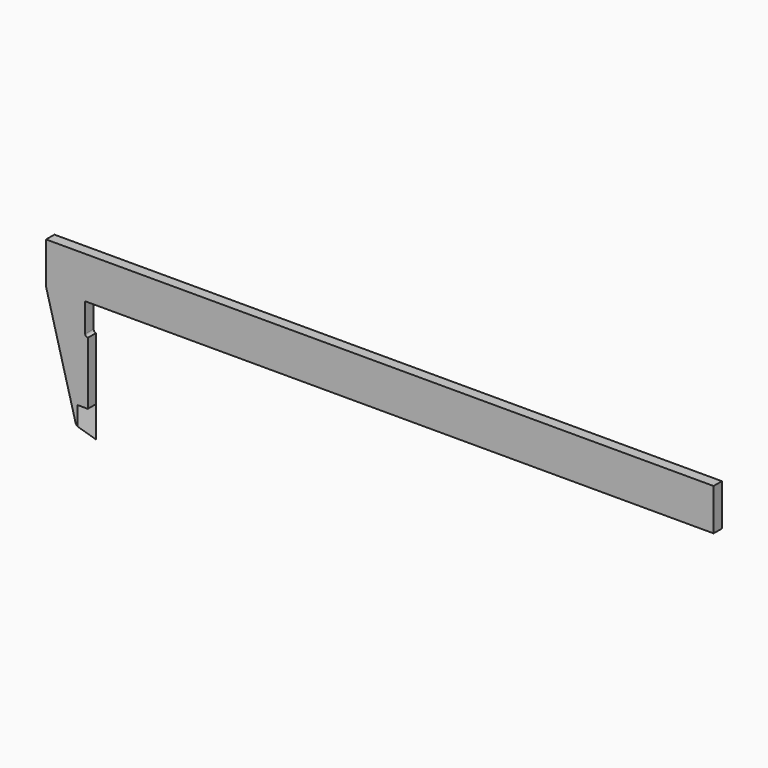
from build123d import *

# Parameters (mm, degrees)
F1_DEPTH = 3.175
F3_DEPTH = 9.525
F5_DEPTH = 3.176


# Not quite as in the source:
# - a feature names something its author has since deleted; it is built from what else it names


with BuildPart() as f1:
    # F0 (on Front) → F1 (new body)
    with BuildSketch(Plane.XZ):
        with BuildLine():
            Line((101.6, 6.35), (-101.6, 6.35))
            Line((-101.6, 6.35), (-101.6, -6.35))
            Line((-101.6, -6.35), (-92.5598257878, -40.0883894691))
            Line((-92.5598257878, -40.0883894691), (-92.075, -40.6661823435))
            Line((-92.075, -40.6661823435), (-92.075, -34.925))
            Line((-92.075, -34.925), (-88.9, -34.925))
            Line((-88.9, -34.925), (-88.9, -15.875))
            ThreePointArc((-88.9, -15.875), (-89.4567758795, -15.6443758795), (-89.6874, -15.0876))
            Line((-89.6874, -15.0876), (-89.6874, -6.35))
            Line((-89.6874, -6.35), (101.6, -6.35))
            Line((101.6, -6.35), (101.6, 6.35))
        make_face()
    extrude(amount=F1_DEPTH)

    # F2 (on face) → F3 (join)
    with BuildSketch(Plane(origin=(0, 0, -34.925), x_dir=(1, 0, 0), z_dir=(0, 0, -1))):
        Polygon((-88.9, 0), (-92.075, 3.175), (-92.075, 0), align=None)
    extrude(amount=F3_DEPTH)

    # F4 (on face) → F5 (cut, through all)
    with BuildSketch(Plane(origin=(0, 0, 0), x_dir=(-1, 0, 0), z_dir=(0, 1, 0))):
        Polygon((92.075, -44.45), (92.075, -40.6661823435), (88.9, -44.45), align=None)
    extrude(amount=-F5_DEPTH, mode=Mode.SUBTRACT)


solid = f1.part
